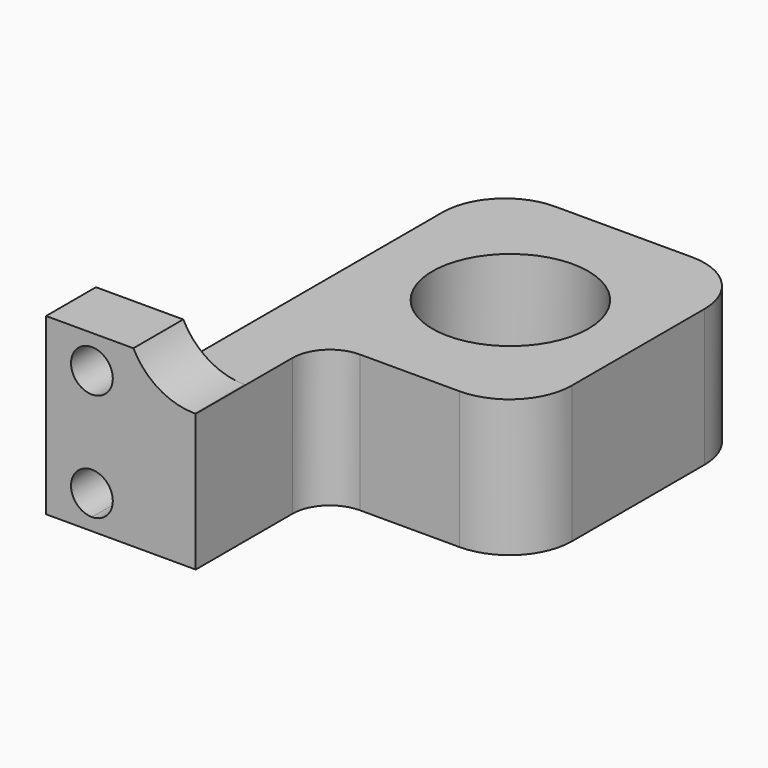
from build123d import *

# Parameters (mm, degrees)
F0_W         = 28
F0_H         = 36
F1_DEPTH     = 4
F2_R         = 6.25
F2_W         = 7
F2_H         = 31
F2_W_2       = 16
F2_H_2       = 12.7
F3_DEPTH     = 25
F4_W         = 7
F4_H         = 5
F4_R         = 6.25
F5_DEPTH     = 7
F6_DEPTH     = 10
F8_DEPTH     = 25
F9_R         = 5
F10_R        = 3
F11_T1_DEPTH = 5


# Not quite as in the source:
# - a fillet or chamfer that OpenCascade refuses, or shapes differently, is made with other operations: its cross-section is extruded or revolved along the edge and cut away or added


with BuildPart() as f1:
    # F0 (on Top) → F1 (new body)
    with BuildSketch(Plane.XY):
        with Locations((14, 18)):
            Rectangle(F0_W, F0_H)
    extrude(amount=F1_DEPTH)

    # F2 (on face) → F3 (cut)
    with BuildSketch(Plane.XY.offset(4)):
        with Locations((17.75, 24.35)):
            Circle(F2_R)
        with Locations((3.5, 20.5)):
            Rectangle(F2_W, F2_H)
        with Locations((20, 6.35)):
            Rectangle(F2_W_2, F2_H_2)
    extrude(amount=-F3_DEPTH, mode=Mode.SUBTRACT)

    # F4 (on face) → F5 (join)
    with BuildSketch(Plane.XY.offset(4)):
        with Locations((3.5, 2.5)):
            Rectangle(F4_W, F4_H)
        Polygon((7, 36), (7, 5), (7, 0), (12, 0), (12, 12.7), (28, 12.7), (28, 36), align=None)
        with Locations((17.75, 24.35)):
            Circle(F4_R, mode=Mode.SUBTRACT)
    extrude(amount=F5_DEPTH)

    # F4 (on face) → F6 (join)
    with BuildSketch(Plane.XY.offset(4)):
        with Locations((3.5, 2.5)):
            Rectangle(F4_W, F4_H)
    extrude(amount=F6_DEPTH)

    # F7 (on face) → F8 (cut)
    with BuildSketch(Plane.XZ):
        with BuildLine():
            ThreePointArc((3.675, 13), (2.4905961415, 10.1405961415), (5.35, 11.325))
            ThreePointArc((5.35, 11.325), (4.8594038585, 12.5094038585), (3.675, 13))
        make_face()
        with BuildLine():
            ThreePointArc((3.675, 1), (4.8594038585, 1.4905961415), (5.35, 2.675))
            ThreePointArc((5.35, 2.675), (2.4905961415, 3.8594038585), (3.675, 1))
        make_face()
    extrude(amount=-F8_DEPTH, mode=Mode.SUBTRACT)

    # F9
    f9_edges = [f1.edges().sort_by_distance(p)[0] for p in [
        (28, 36, 5.5),
        (7, 36, 5.5),
        (28, 12.7, 5.5),
    ]]
    fillet(f9_edges, radius=F9_R)

    # F10
    f10_edges = [f1.edges().sort_by_distance(p)[0] for p in [
        (12, 12.7, 5.5),
    ]]
    fillet(f10_edges, radius=F10_R)

    # F11: fillet of radius 5.5 on 1 edges, made by hand

    # F11_s2 → F11_t1 (join)
    with BuildSketch(Plane.XZ.offset(-5)):
        with BuildLine():
            ThreePointArc((11.8989794856, 11), (9.0266981623, 11.8095842402), (7, 14))
            Line((7, 14), (7, 11))
            Line((7, 11), (11.8989794856, 11))
        make_face()
    extrude(amount=F11_T1_DEPTH)


solid = f1.part
